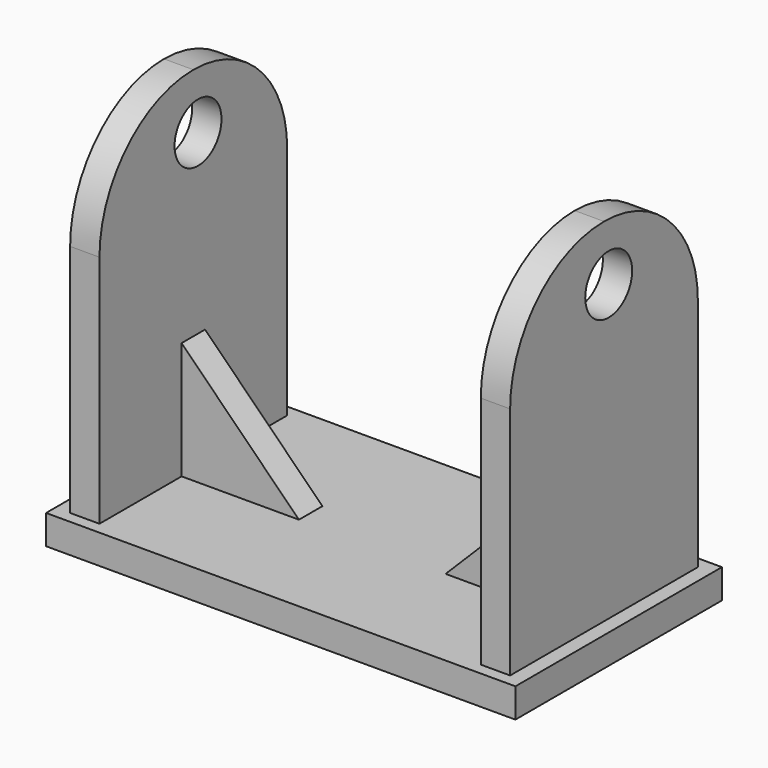
from build123d import *

# Parameters (mm, degrees)
F0_W     = 203.2
F0_H     = 111.76
F1_DEPTH = 12.7
F2_W     = 12.7
F2_H     = 101.6
F3_DEPTH = 152.4
F5_D     = 25.4
F6_R     = 50.79999
F7_R     = 50.79999
F8_W     = 50.8
F8_H     = 12.7
F9_DEPTH = 50.8
F10_SIZE = 50.79999


# Not quite as in the source:
# - a fillet or chamfer is up to 0.001 mm smaller than in the source, because OpenCascade refuses the exact size
# - a feature names something its author has since deleted; it is built from what else it names


with BuildPart() as f1:
    # F0 (on Top) → F1 (new body)
    with BuildSketch(Plane.XY):
        with Locations((0, -2.54)):
            Rectangle(F0_W, F0_H)
    extrude(amount=F1_DEPTH)

    # F2 (on face) → F3 (join)
    with BuildSketch(Plane.XY.offset(12.7)):
        with Locations((-88.9, -2.54)):
            Rectangle(F2_W, F2_H)
        with Locations((88.9, -2.54)):
            Rectangle(F2_W, F2_H)
    extrude(amount=F3_DEPTH)

    # F5 (through all)
    with Locations(Plane.YZ.offset(95.25)):
        with Locations((0, 140.1294022799)):
            Hole(F5_D / 2)

    # F6 (radius 50.8 in the source; OpenCascade refuses exactly that, so slightly less here)
    f6_edges = [f1.edges().sort_by_distance(p)[0] for p in [
        (-88.9, -53.34, 165.1),
        (-88.9, 48.26, 165.1),
    ]]
    fillet(f6_edges, radius=F6_R)

    # F7 (radius 50.8 in the source; OpenCascade refuses exactly that, so slightly less here)
    f7_edges = [f1.edges().sort_by_distance(p)[0] for p in [
        (88.9, -53.34, 165.1),
        (88.9, 48.26, 165.1),
    ]]
    fillet(f7_edges, radius=F7_R)

    # F8 (on face) → F9 (join)
    with BuildSketch(Plane.XY.offset(12.7)):
        with Locations((-57.15, -2.54)):
            Rectangle(F8_W, F8_H)
        with Locations((57.15, -2.54)):
            Rectangle(F8_W, F8_H)
    extrude(amount=F9_DEPTH)

    # F10 (size 50.8 in the source; OpenCascade refuses exactly that, so slightly less here)
    f10_edges = [f1.edges().sort_by_distance(p)[0] for p in [
        (-31.75, -2.54, 63.5),
        (31.75, -2.54, 63.5),
    ]]
    chamfer(f10_edges, length=F10_SIZE)


solid = f1.part
